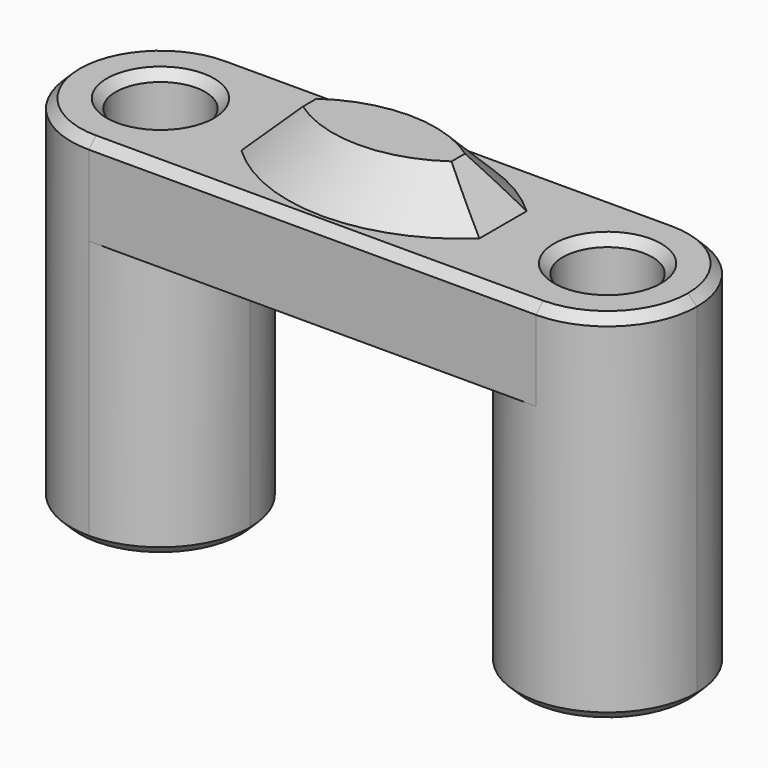
from build123d import *

# Parameters (mm, degrees)
F0_R     = 12.7
F1_DEPTH = 25.4
F2_DEPTH = 76.2
F5_DEPTH = 12.7
F6_SIZE  = 12.69999
F7_SIZE  = 2.54
F8_SIZE  = 2.54
F9_SIZE  = 2.54


# Not quite as in the source:
# - a fillet or chamfer is up to 0.001 mm smaller than in the source, because OpenCascade refuses the exact size


with BuildPart() as f1:
    # F0 (on Top) → F1 (new body)
    with BuildSketch(Plane.XY):
        with BuildLine():
            ThreePointArc((0, -25.4), (17.9605122421, -17.9605122421), (25.4, 0))
            ThreePointArc((25.4, 0), (17.9605122421, 17.9605122421), (0, 25.4))
            ThreePointArc((0, 25.4), (-25.4, 0), (0, -25.4))
        make_face()
        Circle(F0_R, mode=Mode.SUBTRACT)
        with BuildLine():
            ThreePointArc((0, 25.4), (17.9605122421, 17.9605122421), (25.4, 0))
            ThreePointArc((25.4, 0), (17.9605122421, -17.9605122421), (0, -25.4))
            Line((0, -25.4), (127, -25.4))
            ThreePointArc((127, -25.4), (101.6, 0), (127, 25.4))
            Line((127, 25.4), (0, 25.4))
        make_face()
        with BuildLine():
            ThreePointArc((152.4, 0), (144.9605122421, 17.9605122421), (127, 25.4))
            ThreePointArc((127, 25.4), (101.6, 0), (127, -25.4))
            ThreePointArc((127, -25.4), (144.9605122421, -17.9605122421), (152.4, 0))
        make_face()
        with Locations((127, 0)):
            Circle(F0_R, mode=Mode.SUBTRACT)
    extrude(amount=F1_DEPTH)

    # F0 (on Top) → F2 (join)
    with BuildSketch(Plane.XY):
        with BuildLine():
            ThreePointArc((0, -25.4), (17.9605122421, -17.9605122421), (25.4, 0))
            ThreePointArc((25.4, 0), (17.9605122421, 17.9605122421), (0, 25.4))
            ThreePointArc((0, 25.4), (-25.4, 0), (0, -25.4))
        make_face()
        Circle(F0_R, mode=Mode.SUBTRACT)
        with BuildLine():
            ThreePointArc((152.4, 0), (144.9605122421, 17.9605122421), (127, 25.4))
            ThreePointArc((127, 25.4), (101.6, 0), (127, -25.4))
            ThreePointArc((127, -25.4), (144.9605122421, -17.9605122421), (152.4, 0))
        make_face()
        with Locations((127, 0)):
            Circle(F0_R, mode=Mode.SUBTRACT)
    extrude(amount=-F2_DEPTH)

    # F4 (on face) → F5 (join)
    with BuildSketch(Plane.XY.offset(25.4)):
        with BuildLine():
            ThreePointArc((29.6961453219, -8.3886324314), (63.5, -21.7770315987), (97.3038546781, -8.3886324314))
            Line((97.3038546781, -8.3886324314), (97.3038546781, 8.3886324314))
            ThreePointArc((97.3038546781, 8.3886324314), (63.5, 21.7770315987), (29.6961453219, 8.3886324314))
            Line((29.6961453219, 8.3886324314), (29.6961453219, -8.3886324314))
        make_face()
    extrude(amount=F5_DEPTH)

    # F6 (size 12.7 in the source; OpenCascade refuses exactly that, so slightly less here)
    f6_edges = [f1.edges().sort_by_distance(p)[0] for p in [
        (63.5, -21.777032, 38.1),
        (97.303855, 0, 38.1),
        (63.5, 21.777032, 38.1),
        (29.696145, 0, 38.1),
    ]]
    chamfer(f6_edges, length=F6_SIZE)

    # F7
    f7_edges = [f1.edges().sort_by_distance(p)[0] for p in [
        (114.3, 0, 25.4),
        (-12.7, 0, 25.4),
    ]]
    chamfer(f7_edges, length=F7_SIZE)

    # F8
    f8_edges = [f1.edges().sort_by_distance(p)[0] for p in [
        (114.3, 0, -76.2),
        (127, -25.4, -76.2),
        (-25.4, 0, -76.2),
        (-12.7, 0, -76.2),
    ]]
    chamfer(f8_edges, length=F8_SIZE)

    # F9
    f9_edges = [f1.edges().sort_by_distance(p)[0] for p in [
        (63.5, -25.4, 25.4),
    ]]
    chamfer(f9_edges, length=F9_SIZE)


solid = f1.part
